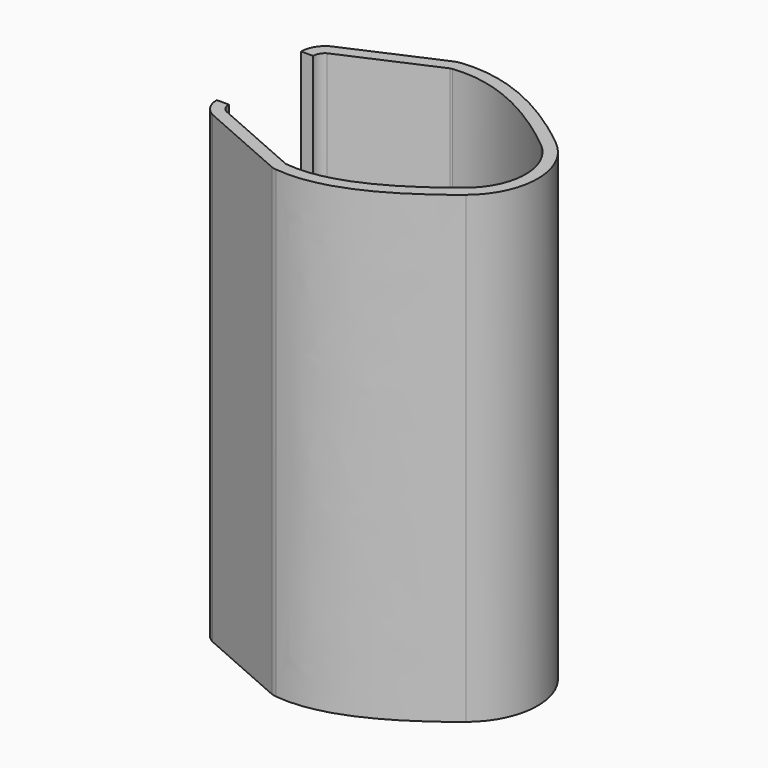
from build123d import *

# Parameters (mm, degrees)
F1_DEPTH = 96
F2_T     = 2.5


# Not quite as in the source:
# - a shell that OpenCascade refuses in one call is made with other operations: the cavity is built on its own and cut out


with BuildPart() as f1:
    # F0 (on Top) → F1 (new body)
    with BuildSketch(Plane.XY):
        with BuildLine():
            Line((-23.4862479759, 10.9015624084), (-23.4862479759, 0))
            Line((-23.4862479759, 0), (-23.4862479759, -10.9015624084))
            ThreePointArc((-23.4862479759, -10.9015624084), (-22.7949669389, -13.4382809378), (-20.9122716169, -15.273565301))
            Line((-20.9122716169, -15.273565301), (-1.9122716169, -23.6296655884))
            ThreePointArc((-1.9122716169, -23.6296655884), (-1.3870055148, -23.7814630999), (-0.8483054026, -23.875))
            add(Edge.make_bspline(
                [(-0.8483054026, -23.875), (9.4434290002, -25.0869225879), (20.0678939818, -18.6179530115), (28.6502054798, -11.6355601057)],
                knots=[0, 0, 0, 0, 30.2768962954, 30.2768962954, 30.2768962954, 30.2768962954], degree=3))
            ThreePointArc((28.6502054798, -11.6355601057), (34.1837520241, 0), (28.6502054798, 11.6355601057))
            add(Edge.make_bspline(
                [(-0.8483054026, 23.875), (9.4434290002, 25.0869225879), (20.0678939818, 18.6179530115), (28.6502054798, 11.6355601057)],
                knots=[0, 0, 0, 0, 30.2768962954, 30.2768962954, 30.2768962954, 30.2768962954], degree=3))
            ThreePointArc((-0.8483054026, 23.875), (-1.3870055148, 23.7814630999), (-1.9122716169, 23.6296655884))
            Line((-1.9122716169, 23.6296655884), (-20.9122716169, 15.273565301))
            ThreePointArc((-20.9122716169, 15.273565301), (-22.7949669389, 13.4382809378), (-23.4862479759, 10.9015624084))
        make_face()
    extrude(amount=F1_DEPTH)

    # F2: shell of thickness 2.5, made by hand


with BuildPart() as f2_core1:
    # F2_t2: copy of F1
    add(f1.part)

    # the walls: a layer under each face that stays
    f2_faces = [f2_core1.faces().sort_by_distance(p)[0] for p in [
        (-11.4122716169, 19.4516154447, 48),
        (14.5419836279, 20.828148363, 48),
        (34.1837520241, 0, 48),
        (14.5419836279, -20.828148363, 48),
        (-1.3870055148, -23.7814630999, 48),
        (-11.4122716169, -19.4516154447, 48),
        (-22.7949669389, -13.4382809378, 48),
        (5.3487520241, 0, 0),
        (-22.7949669389, 13.4382809378, 48),
        (-1.3870055148, 23.7814630999, 48),
    ]]
    thicken(f2_faces, amount=-F2_T, mode=Mode.SUBTRACT)


with BuildPart() as f1_1:
    add(f1.part)

    # what is left inside the walls is the cavity
    f2_cavity = [f2_core1.part.solids().sort_by_distance(p)[0] for p in [
        (13.474931, 18.539694, 64.833333),
    ]]
    add(f2_cavity, mode=Mode.SUBTRACT)


solid = f1_1.part
